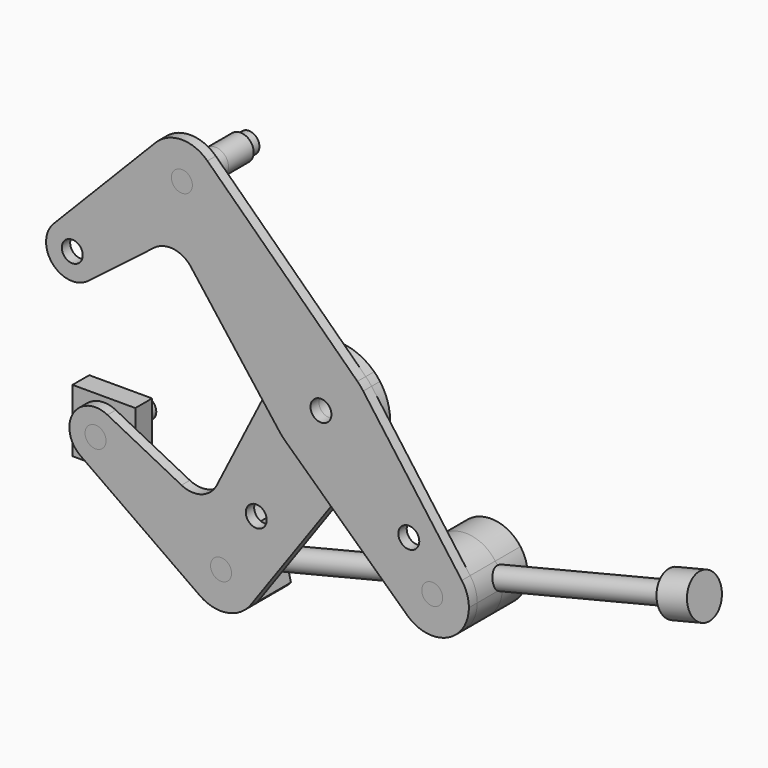
from build123d import *

# Parameters (mm, degrees)
F0_R      = 3.175
F0_R_2    = 3.9751
F1_DEPTH  = 3.175
F2_DEPTH  = 3.175
F3_R      = 3.175
F6_DEPTH  = 12.7
F3_R_2    = 3.9751
F4_R      = 3.9751
F4_R_2    = 3.175
F11_R     = 3.175
F12_DEPTH = 12.7
F13_DEPTH = 127
F14_R     = 6.35
F14_R_2   = 3.175
F15_DEPTH = 9.525
F16_R     = 3.175
F17_DEPTH = 6.35


with BuildPart() as f1:
    # F0 (on Front) → F1 (new body)
    with BuildSketch(Plane.XZ):
        with BuildLine():
            Line((-1.7976106712, -14.3453010855), (-7.8255865168, -6.4334713683))
            Line((-7.8255865168, -6.4334713683), (-23.2839574438, -36.9892948112))
            ThreePointArc((-23.2839574438, -36.9892948112), (-27.9130287782, -40.9587935194), (-33.99229114, -40.481519439))
            Line((-33.99229114, -40.481519439), (-56.4423916697, -29.0227267269))
            ThreePointArc((-56.4423916697, -29.0227267269), (-53.2816250221, -31.9476026962), (-52.1134142985, -36.0925549206))
            ThreePointArc((-52.1134142985, -36.0925549206), (-56.4000701161, -43.1406215353), (-64.6300109614, -42.5760555184))
            Line((-64.6300109614, -42.5760555184), (-28.4151474925, -68.1534975119))
            ThreePointArc((-28.4151474925, -68.1534975119), (-27.1155940199, -49.2093034143), (-10.8919121645, -59.0765966749))
            ThreePointArc((-10.8919121645, -59.0765966749), (-11.4190694743, -62.458633987), (-12.9505265861, -65.5197955841))
            Line((-12.9505265861, -65.5197955841), (13.2537806818, -28.697899658))
            Line((13.2537806818, -28.697899658), (0, -16.3316972949))
            ThreePointArc((0, -16.3316972949), (-0.9407825859, -15.3764869555), (-1.7976106712, -14.3453010855))
        make_face()
        with Locations((-11.3266830524, -41.4012788264)):
            Circle(F0_R, mode=Mode.SUBTRACT)
        with BuildLine():
            Line((-3.3354770071, 2.4419136296), (-7.8255865168, -6.4334713683))
            Line((-7.8255865168, -6.4334713683), (-1.7976106712, -14.3453010855))
            ThreePointArc((-1.7976106712, -14.3453010855), (-4.9788694599, -6.172685383), (-3.3354770071, 2.4419136296))
        make_face()
        with BuildLine():
            ThreePointArc((23.6362700176, 4.6570929355), (22.798996702, 5.7042185542), (21.876354173, 6.676961804))
            ThreePointArc((21.876354173, 6.676961804), (8.2001172895, 10.9312093345), (-3.3354770071, 2.4419136296))
            ThreePointArc((-3.3354770071, 2.4419136296), (-4.9788694599, -6.172685383), (-1.7976106712, -14.3453010855))
            ThreePointArc((-1.7976106712, -14.3453010855), (-0.9407825859, -15.3764869555), (0, -16.3316972949))
            ThreePointArc((0, -16.3316972949), (12.4268416726, -20.5189279155), (23.7640554537, -13.9290206394))
            ThreePointArc((23.7640554537, -13.9290206394), (25.9518513278, -9.5559326435), (26.7049331988, -4.7244507692))
            ThreePointArc((26.7049331988, -4.7244507692), (25.9182767461, 0.2108824517), (23.6362700176, 4.6570929355))
        make_face()
        with Locations((10.8299331988, -4.7244507692)):
            Circle(F0_R_2, mode=Mode.SUBTRACT)
        with BuildLine():
            ThreePointArc((23.7640554537, -13.9290206394), (12.4268416726, -20.5189279155), (0, -16.3316972949))
            Line((0, -16.3316972949), (13.2537806818, -28.697899658))
            Line((13.2537806818, -28.697899658), (23.7640554537, -13.9290206394))
        make_face()
        with BuildLine():
            ThreePointArc((-52.1134142985, -36.0925549206), (-53.2816250221, -31.9476026962), (-56.4423916697, -29.0227267269))
            ThreePointArc((-56.4423916697, -29.0227267269), (-66.8449325368, -31.9882617501), (-64.6300109614, -42.5760555184))
            ThreePointArc((-64.6300109614, -42.5760555184), (-56.4000701161, -43.1406215353), (-52.1134142985, -36.0925549206))
        make_face()
        with Locations((-60.0509142985, -36.0925549206)):
            Circle(F0_R, mode=Mode.SUBTRACT)
        with BuildLine():
            ThreePointArc((-28.4151474925, -68.1534975119), (-20.1387601947, -70.0313672785), (-12.9505265861, -65.5197955841))
            ThreePointArc((-12.9505265861, -65.5197955841), (-11.4190694743, -62.458633987), (-10.8919121645, -59.0765966749))
            ThreePointArc((-10.8919121645, -59.0765966749), (-27.1155940199, -49.2093034143), (-28.4151474925, -68.1534975119))
        make_face()
        with Locations((-22.0044121645, -59.0765966749)):
            Circle(F0_R, mode=Mode.SUBTRACT)
        with Locations((10.8299331988, -4.7244507692)):
            Circle(F0_R_2)
        with Locations((10.8299331988, -4.7244507692)):
            Circle(F0_R, mode=Mode.SUBTRACT)
    extrude(amount=-F1_DEPTH)


with BuildPart() as f2:
    # F0 (on Front) → F2 (new body)
    with BuildSketch(Plane.XZ):
        with BuildLine():
            ThreePointArc((-70.251397086, 18.7865048472), (-61.5778622997, 20.594649096), (-56.6330061539, 13.2429153541))
            ThreePointArc((-56.6330061539, 13.2429153541), (-57.4513110928, 9.7327917193), (-59.7375020108, 6.9464101963))
            Line((-59.7375020108, 6.9464101963), (-39.743073588, 22.2935199))
            ThreePointArc((-39.743073588, 22.2935199), (-33.8517175555, 23.8674149125), (-28.5784626681, 20.8050621724))
            Line((-28.5784626681, 20.8050621724), (-7.8255865168, -6.4334713683))
            Line((-7.8255865168, -6.4334713683), (-3.3354770071, 2.4419136296))
            ThreePointArc((-3.3354770071, 2.4419136296), (8.2001172895, 10.9312093345), (21.876354173, 6.676961804))
            Line((21.876354173, 6.676961804), (-23.6008493451, 50.7381982134))
            ThreePointArc((-23.6008493451, 50.7381982134), (-21.1006756701, 47.0908169797), (-20.220844027, 42.7572094122))
            ThreePointArc((-20.220844027, 42.7572094122), (-35.5230454229, 32.4647821735), (-39.2865913319, 50.5182347025))
            Line((-39.2865913319, 50.5182347025), (-70.251397086, 18.7865048472))
        make_face()
        with BuildLine():
            ThreePointArc((-59.7375020108, 6.9464101963), (-57.4513110928, 9.7327917193), (-56.6330061539, 13.2429153541))
            ThreePointArc((-56.6330061539, 13.2429153541), (-61.5778622997, 20.594649096), (-70.251397086, 18.7865048472))
            ThreePointArc((-70.251397086, 18.7865048472), (-70.5057136766, 7.9725057009), (-59.7375020108, 6.9464101963))
        make_face()
        with Locations((-64.5705061539, 13.2429153541)):
            Circle(F0_R, mode=Mode.SUBTRACT)
        with BuildLine():
            ThreePointArc((-23.6008493451, 50.7381982134), (-31.4891609602, 53.8686169438), (-39.2865913319, 50.5182347025))
            ThreePointArc((-39.2865913319, 50.5182347025), (-35.5230454229, 32.4647821735), (-20.220844027, 42.7572094122))
            ThreePointArc((-20.220844027, 42.7572094122), (-21.1006756701, 47.0908169797), (-23.6008493451, 50.7381982134))
        make_face()
        with Locations((-31.333344027, 42.7572094122)):
            Circle(F0_R, mode=Mode.SUBTRACT)
        with BuildLine():
            ThreePointArc((23.6362700176, 4.6570929355), (22.798996702, 5.7042185542), (21.876354173, 6.676961804))
            ThreePointArc((21.876354173, 6.676961804), (8.2001172895, 10.9312093345), (-3.3354770071, 2.4419136296))
            ThreePointArc((-3.3354770071, 2.4419136296), (-4.9788694599, -6.172685383), (-1.7976106712, -14.3453010855))
            ThreePointArc((-1.7976106712, -14.3453010855), (-0.9407825859, -15.3764869555), (0, -16.3316972949))
            ThreePointArc((0, -16.3316972949), (12.4268416726, -20.5189279155), (23.7640554537, -13.9290206394))
            ThreePointArc((23.7640554537, -13.9290206394), (25.9518513278, -9.5559326435), (26.7049331988, -4.7244507692))
            ThreePointArc((26.7049331988, -4.7244507692), (25.9182767461, 0.2108824517), (23.6362700176, 4.6570929355))
        make_face()
        with Locations((10.8299331988, -4.7244507692)):
            Circle(F0_R_2, mode=Mode.SUBTRACT)
        with BuildLine():
            Line((-3.3354770071, 2.4419136296), (-7.8255865168, -6.4334713683))
            Line((-7.8255865168, -6.4334713683), (-1.7976106712, -14.3453010855))
            ThreePointArc((-1.7976106712, -14.3453010855), (-4.9788694599, -6.172685383), (-3.3354770071, 2.4419136296))
        make_face()
        with BuildLine():
            ThreePointArc((23.7640554537, -13.9290206394), (12.4268416726, -20.5189279155), (0, -16.3316972949))
            Line((0, -16.3316972949), (13.2537806818, -28.697899658))
            Line((13.2537806818, -28.697899658), (23.7640554537, -13.9290206394))
        make_face()
        with Locations((10.8299331988, -4.7244507692)):
            Circle(F0_R_2)
        with Locations((10.8299331988, -4.7244507692)):
            Circle(F0_R, mode=Mode.SUBTRACT)
        with BuildLine():
            Line((53.5249907527, -36.142698321), (23.6362700176, 4.6570929355))
            ThreePointArc((23.6362700176, 4.6570929355), (25.9182767461, 0.2108824517), (26.7049331988, -4.7244507692))
            ThreePointArc((26.7049331988, -4.7244507692), (25.9518513278, -9.5559326435), (23.7640554537, -13.9290206394))
            Line((23.7640554537, -13.9290206394), (13.2537806818, -28.697899658))
            Line((13.2537806818, -28.697899658), (36.9796017403, -50.8348514823))
            ThreePointArc((36.9796017403, -50.8348514823), (37.181981465, -34.4004883825), (53.5249907527, -36.142698321))
        make_face()
        with Locations((37.4563332682, -29.9277378442)):
            Circle(F0_R, mode=Mode.SUBTRACT)
        with BuildLine():
            ThreePointArc((55.6730549795, -42.7097789143), (55.1223954626, -39.2550456597), (53.5249907527, -36.142698321))
            ThreePointArc((53.5249907527, -36.142698321), (37.181981465, -34.4004883825), (36.9796017403, -50.8348514823))
            ThreePointArc((36.9796017403, -50.8348514823), (48.99024534, -52.9012213814), (55.6730549795, -42.7097789143))
        make_face()
        with Locations((44.5605549795, -42.7097789143)):
            Circle(F0_R, mode=Mode.SUBTRACT)
    extrude(amount=F2_DEPTH)


with BuildPart() as f6:
    # F3 (on face) → F6 (new body, through all)
    with BuildSketch(Plane.XZ.offset(3.175)):
        with BuildLine():
            ThreePointArc((36.9796017403, -50.8348514823), (48.99024534, -52.9012213814), (55.6730549795, -42.7097789143))
            ThreePointArc((55.6730549795, -42.7097789143), (55.1223954626, -39.2550456597), (53.5249907527, -36.142698321))
            ThreePointArc((53.5249907527, -36.142698321), (37.181981465, -34.4004883825), (36.9796017403, -50.8348514823))
        make_face()
        with Locations((44.5605549795, -42.7097789143)):
            Circle(F3_R, mode=Mode.SUBTRACT)
        with Locations((44.5605549795, -42.7097789143)):
            Circle(F3_R)
    extrude(amount=-F6_DEPTH)

    # F7: cut F2
    add(f2.part, mode=Mode.SUBTRACT)


with BuildPart() as f6b:
    # F3 (on face) → F6, piece 2 (new body, through all)
    with BuildSketch(Plane.XZ.offset(3.175)):
        with Locations((-31.333344027, 42.7572094122)):
            Circle(F3_R_2)
        with Locations((-31.333344027, 42.7572094122)):
            Circle(F3_R, mode=Mode.SUBTRACT)
        with Locations((-31.333344027, 42.7572094122)):
            Circle(F3_R)
    extrude(amount=-F6_DEPTH)

    # F7: cut F2
    add(f2.part, mode=Mode.SUBTRACT)


with BuildPart() as f6c:
    # F4 (on Front) → F6, piece 3 (new body, through all)
    with BuildSketch(Plane.XZ):
        with Locations((-60.0509142985, -36.0925549206)):
            Circle(F4_R)
        with Locations((-60.0509142985, -36.0925549206)):
            Circle(F4_R_2, mode=Mode.SUBTRACT)
        with Locations((-60.0509142985, -36.0925549206)):
            Circle(F4_R_2)
    extrude(amount=-F6_DEPTH)

    # F8: cut F1
    add(f1.part, mode=Mode.SUBTRACT)


with BuildPart() as f6d:
    # F4 (on Front) → F6, piece 4 (new body, through all)
    with BuildSketch(Plane.XZ):
        with BuildLine():
            Line((-15.6544121645, -57.5152754989), (-17.7996864895, -48.7902981061))
            ThreePointArc((-17.7996864895, -48.7902981061), (-32.7955071278, -61.729882514), (-13.5091378396, -66.2402528918))
            Line((-13.5091378396, -66.2402528918), (-15.6544121645, -57.5152754989))
        make_face()
        with Locations((-22.0044121645, -59.0765966749)):
            Circle(F4_R_2, mode=Mode.SUBTRACT)
        with Locations((-22.0044121645, -59.0765966749)):
            Circle(F4_R_2)
    extrude(amount=-F6_DEPTH)

    # F8: cut F1
    add(f1.part, mode=Mode.SUBTRACT)


with BuildPart() as f9_1:
    # F9: instance of F6b
    add(f6b.part.mirror(Plane.XZ.offset(-9.525)))


with BuildPart() as f9_2:
    # F9: instance of F6
    add(f6.part.mirror(Plane.XZ.offset(-9.525)))


with BuildPart() as f9_3:
    # F9: instance of F6d
    add(f6d.part.mirror(Plane.XZ.offset(-9.525)))


with BuildPart() as f9_4:
    # F9: instance of F6c
    add(f6c.part.mirror(Plane.XZ.offset(-9.525)))


with BuildPart() as f6b_1:
    add(f6b.part)

    # F10: union F9_1, F6, F6c, F6d, F9_2, F9_4, F9_3
    add(f9_1.part)
    add(f6.part)
    add(f6c.part)
    add(f6d.part)
    add(f9_2.part)
    add(f9_4.part)
    add(f9_3.part)


with BuildPart() as f12:
    # F11 (on face) → F12 (new body)
    with BuildSketch(Plane(origin=(-28.0974646283, 0, -6.9085301599), x_dir=(0, 1, 0), z_dir=(0.971077162, 0, 0.2387658798))):
        with Locations((9.525, -52.114031013)):
            Circle(F11_R)
    extrude(amount=-F12_DEPTH)

    # F13 (add): a face of the model
    f13_faces = [f12.faces().sort_by_distance(p)[0] for p in [
        (-15.6544121645, 9.525, -57.5152754989),
    ]]
    extrude(f13_faces, amount=F13_DEPTH)

    # F14 (on face) → F15 (join)
    with BuildSketch(Plane(origin=(95.2293349518, 0, 23.4147365724), x_dir=(0, 1, 0), z_dir=(0.971077162, 0, 0.2387658798))):
        with Locations((9.525, -52.114031013)):
            Circle(F14_R)
        with Locations((9.525, -52.114031013)):
            Circle(F14_R_2, mode=Mode.SUBTRACT)
        with Locations((9.525, -52.114031013)):
            Circle(F14_R_2)
    extrude(amount=F15_DEPTH)


with BuildPart() as f17:
    # F16 (on face) → F17 (new body, through all)
    with BuildSketch(Plane(origin=(0, 3.175, 0), x_dir=(-1, 0, 0), z_dir=(0, 1, 0))):
        with BuildLine():
            Line((69.5759142985, -45.6175549206), (69.5759142985, -26.5675549206))
            Line((69.5759142985, -26.5675549206), (50.5259142985, -26.5675549206))
            Line((50.5259142985, -26.5675549206), (50.5259142985, -32.0425656667))
            Line((50.5259142985, -32.0425656667), (56.4423916697, -29.0227267269))
            ThreePointArc((56.4423916697, -29.0227267269), (66.8449325368, -31.9882617501), (64.6300109614, -42.5760555184))
            Line((64.6300109614, -42.5760555184), (60.3235800987, -45.6175549206))
            Line((60.3235800987, -45.6175549206), (69.5759142985, -45.6175549206))
        make_face()
        with BuildLine():
            Line((56.4423916697, -29.0227267269), (50.5259142985, -32.0425656667))
            Line((50.5259142985, -32.0425656667), (50.5259142985, -45.6175549206))
            Line((50.5259142985, -45.6175549206), (60.3235800987, -45.6175549206))
            Line((60.3235800987, -45.6175549206), (64.6300109614, -42.5760555184))
            ThreePointArc((64.6300109614, -42.5760555184), (66.8449325368, -31.9882617501), (56.4423916697, -29.0227267269))
        make_face()
        with Locations((60.0509142985, -36.0925549206)):
            Circle(F16_R, mode=Mode.SUBTRACT)
    extrude(amount=F17_DEPTH)


solid = Compound([f1.part, f2.part, f6b_1.part, f12.part, f17.part])
